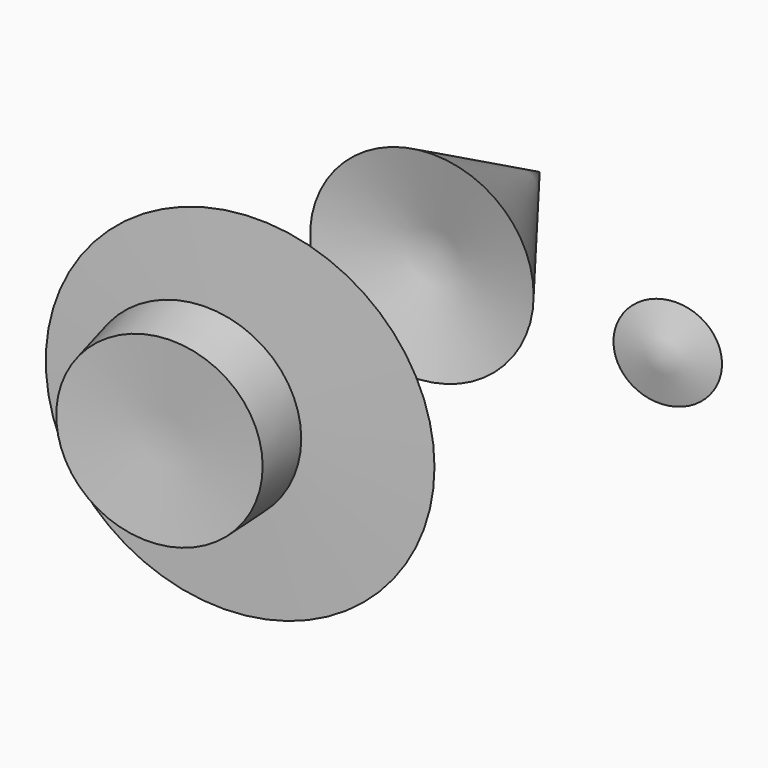
from build123d import *


# Not quite as in the source:
# - the program builds the solid bodies; features that only make, move or delete a surface that nothing else refers to are left out


with BuildPart() as f1:
    # F0 (on Top) → F1 (revolve)
    with BuildSketch(Plane.XY):
        Polygon((-3.8136900403, 31.637430191), (-35.5775393546, 73.2222646475), (-29.7104893918, 33.8516127608), align=None)
    revolve(axis=Axis((-24.3563177064, -2.0773857832, 0), (0.147393288, -0.9890779639, 0)))


with BuildPart() as f5:
    # F4 (on Top) → F5 (revolve)
    with BuildSketch(Plane.XY):
        Polygon((26.3807494193, -37.1444262564), (-22.0485106111, -9.9326465279), (-17.1690713614, -44.4780178368), align=None)
    revolve(axis=Axis((-19.6087909862, -27.2053321823, 0), (0.1398590071, -0.9901714287, 0)))


with BuildPart() as f7:
    # F6 (on Top) → F7 (revolve)
    with BuildSketch(Plane.XY):
        Polygon((-1.4348968238, -44.0676359677), (-25.4218969494, -46.3112071157), (-22.85999991, -60.303106904), (0, -57.9382739961), align=None)
    revolve(axis=Axis((-24.1409484297, -53.3071570098, 0), (0.1801044624, -0.983647489, 0)))


with BuildPart() as f9:
    # F8 (on Top) → F9 (revolve)
    with BuildSketch(Plane.XY):
        Polygon((29.9544837326, 36.2606905401), (24.8306915164, 36.2606905401), (20.49517259, 26.2101721019), (32.5163789093, 26.2101721019), align=None)
    revolve(axis=Axis((31.235431321, 31.235431321, 0), (0.247003553, -0.9690145741, 0)))


solid = Compound([f1.part, f5.part, f7.part, f9.part])
